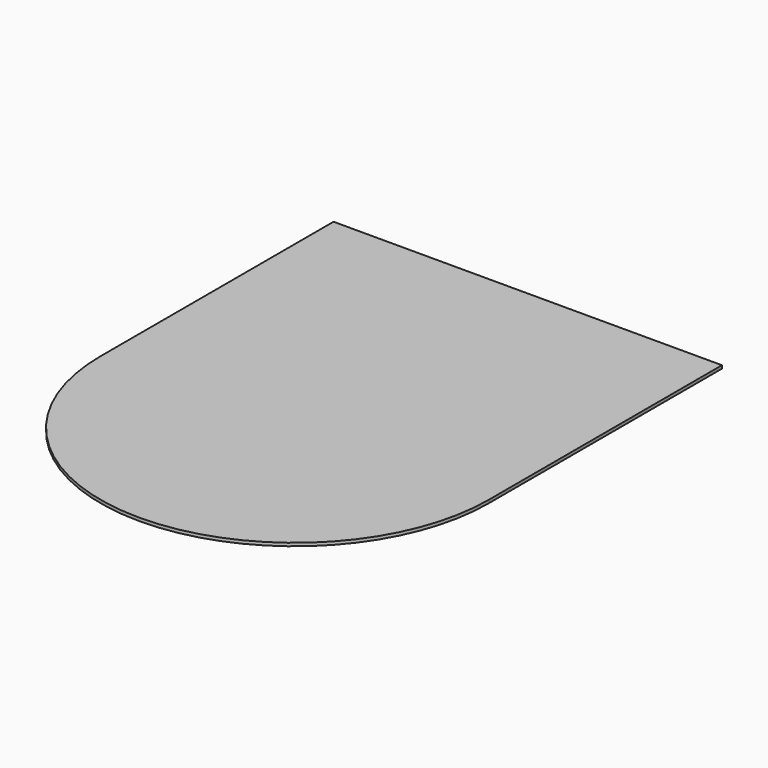
from build123d import *

# Parameters (mm, degrees)
F1_DEPTH = 3.175


with BuildPart() as f1:
    # F0 (on Top) → F1 (new body)
    with BuildSketch(Plane.XY):
        with BuildLine():
            ThreePointArc((-200, 0), (-141.4213562373, 141.4213562373), (0, 200))
            Line((0, 200), (0, 300))
            Line((0, 300), (-200, 300))
            Line((-200, 300), (-200, 0))
        make_face()
        with BuildLine():
            Line((0, 300), (0, 200))
            ThreePointArc((0, 200), (141.4213562373, 141.4213562373), (200, 0))
            Line((200, 0), (200, 300))
            Line((200, 300), (0, 300))
        make_face()
        with BuildLine():
            Line((-200, 0), (0, 0))
            Line((0, 0), (0, 200))
            ThreePointArc((0, 200), (-141.4213562373, 141.4213562373), (-200, 0))
        make_face()
        with BuildLine():
            Line((0, 200), (0, 0))
            Line((0, 0), (-200, 0))
            ThreePointArc((-200, 0), (0, -200), (200, 0))
            ThreePointArc((200, 0), (141.4213562373, 141.4213562373), (0, 200))
        make_face()
    extrude(amount=F1_DEPTH)


solid = f1.part
